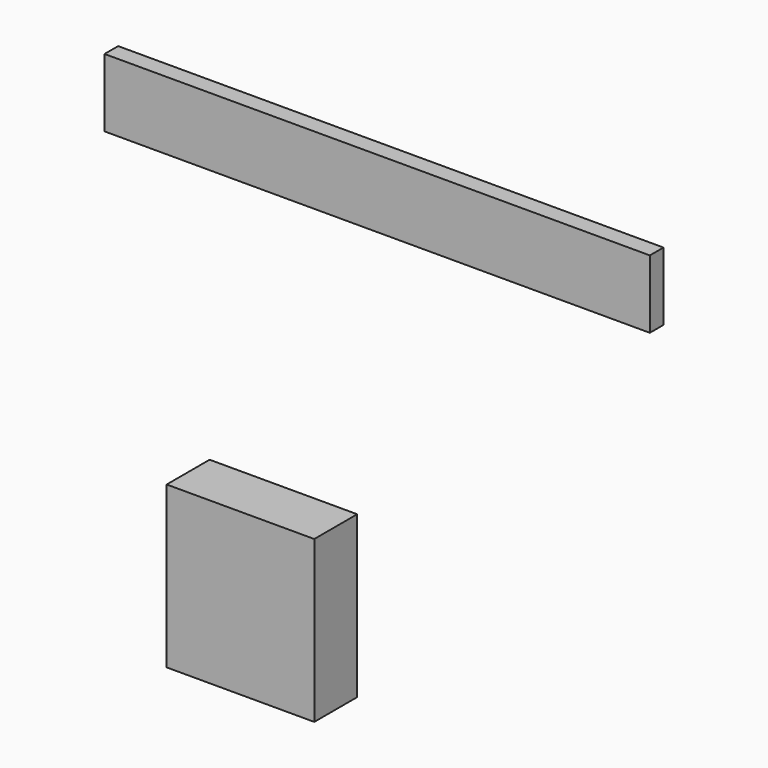
from build123d import *

# Parameters (mm, degrees)
F0_W     = 101.6
F0_H     = 12.7
F1_DEPTH = 3.175
F2_W     = 10
F2_H     = 30
F3_DEPTH = 27.5


# Not quite as in the source:
# - a length typed as a fraction of an inch, garbled in the dataset ("3 / 203.2 mm" for 3/8 in), is restored


with BuildPart() as f1:
    # F0 (on Front) → F1 (new body)
    with BuildSketch(Plane.XZ):
        with Locations((9.3306104093, -6.35)):
            Rectangle(F0_W, F0_H)
    extrude(amount=F1_DEPTH)


with BuildPart() as f3:
    # F2 (on Right) → F3 (new body)
    with BuildSketch(Plane.YZ):
        with Locations((-35.5390549273, -56.9397062063)):
            Rectangle(F2_W, F2_H)
    extrude(amount=F3_DEPTH)


solid = Compound([f1.part, f3.part])
